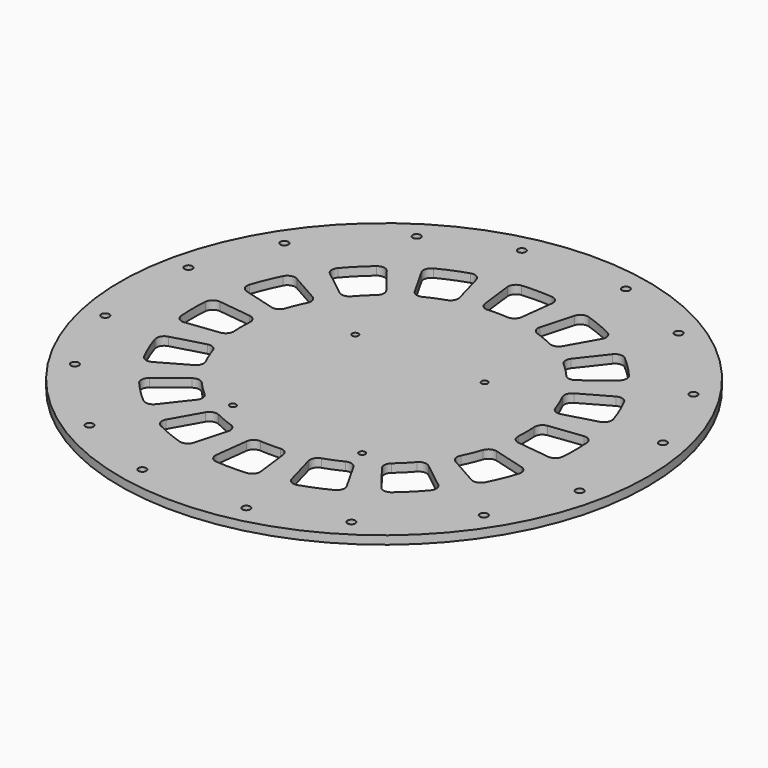
from build123d import *

# Parameters (mm, degrees)
F0_R            = 100
F1_DEPTH        = 3.175
F2_R            = 1.5
F3_DEPTH        = 3.176
F4_R            = 1.2
F5_DEPTH        = 3.176
F7_DEPTH        = 3.176
F7_COPIES_COUNT = 16


# Not quite as in the source:
# - a pattern or mirror of a feature is missing from the dataset's text; its kind, count and spacing are read off the source's solid


with BuildPart() as f1:
    # F0 (on Top) → F1 (new body)
    with BuildSketch(Plane.XY):
        Circle(F0_R)
    extrude(amount=F1_DEPTH)

    # F2 (on face) → F3 (cut, through all)
    with BuildSketch(Plane.XY.offset(3.175)):
        with Locations((19.7, -89.8660670109)):
            Circle(F2_R)
        with Locations((-19.7, -89.8660670109)):
            Circle(F2_R)
        with Locations((-49.6149017926, -77.4749089713)):
            Circle(F2_R)
        with Locations((-77.4749089713, -49.6149017926)):
            Circle(F2_R)
        with Locations((-89.8660670109, -19.7)):
            Circle(F2_R)
        with Locations((-89.8660670109, 19.7)):
            Circle(F2_R)
        with Locations((-77.4749089713, 49.6149017926)):
            Circle(F2_R)
        with Locations((-49.6149017926, 77.4749089713)):
            Circle(F2_R)
        with Locations((-19.7, 89.8660670109)):
            Circle(F2_R)
        with Locations((19.7, 89.8660670109)):
            Circle(F2_R)
        with Locations((49.6149017926, 77.4749089713)):
            Circle(F2_R)
        with Locations((77.4749089713, 49.6149017926)):
            Circle(F2_R)
        with Locations((89.8660670109, 19.7)):
            Circle(F2_R)
        with Locations((89.8660670109, -19.7)):
            Circle(F2_R)
        with Locations((77.4749089713, -49.6149017926)):
            Circle(F2_R)
        with Locations((49.6149017926, -77.4749089713)):
            Circle(F2_R)
    extrude(amount=-F3_DEPTH, mode=Mode.SUBTRACT)

    # F4 (on face) → F5 (cut, through all)
    with BuildSketch(Plane.XY.offset(3.175)):
        with Locations((24.5, 17)):
            Circle(F4_R)
        with Locations((24.5, -41)):
            Circle(F4_R)
        with Locations((-24.5, -41)):
            Circle(F4_R)
        with Locations((-24.5, 17)):
            Circle(F4_R)
    extrude(amount=-F5_DEPTH, mode=Mode.SUBTRACT)

    # F6 (on face) → F7 (cut, through all)
    with BuildSketch(Plane.XY.offset(3.175)):
        with BuildLine():
            Line((-6.9287601414, -56.459818003), (-8.4576550719, -68.9181983999))
            ThreePointArc((-8.4576550719, -68.9181983999), (-7.8034821932, -71.1813531277), (-5.7165399208, -72.2742773837))
            ThreePointArc((-5.7165399208, -72.2742773837), (0, -72.5), (5.7165399208, -72.2742773837))
            ThreePointArc((5.7165399208, -72.2742773837), (7.8034821932, -71.1813531277), (8.4576550719, -68.9181983999))
            Line((8.4576550719, -68.9181983999), (6.9287601414, -56.459818003))
            ThreePointArc((6.9287601414, -56.459818003), (5.8598627663, -54.5108001488), (3.7430088117, -53.8324628217))
            ThreePointArc((3.7430088117, -53.8324628217), (0, -53.9624329364), (-3.7430088117, -53.8324628217))
            ThreePointArc((-3.7430088117, -53.8324628217), (-5.8598627663, -54.5108001488), (-6.9287601414, -56.459818003))
        make_face()
    f7 = extrude(amount=-F7_DEPTH, mode=Mode.SUBTRACT)

    # F7_copies: F7 ×16 about axis
    f7_copies_axis = Axis((0, 0, 0), (0, 0, 1))
    for i in range(1, F7_COPIES_COUNT):
        add(f7.rotate(f7_copies_axis, i * 360 / F7_COPIES_COUNT), mode=Mode.SUBTRACT)


solid = f1.part
